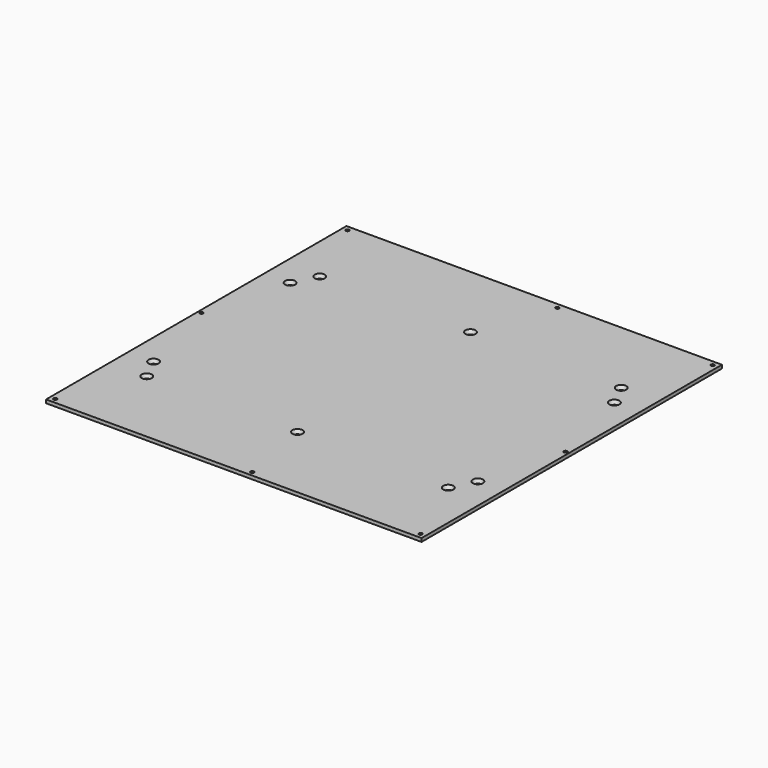
from build123d import *

# Parameters (mm, degrees)
F0_W       = 330
F0_H       = 330
F0_R       = 1.5
F0_R_2     = 2.6
F1_DEPTH   = 3
F2_SIZE2   = 1.849213
F2_SIZE    = 2.99999
F3_SIZE2   = 1.849213
F3_SIZE    = 2.99999
F3_2_SIZE2 = 1.849213
F3_2_SIZE  = 2.99999
F3_3_SIZE2 = 1.849213
F3_3_SIZE  = 2.99999
F3_4_SIZE2 = 1.849213
F3_4_SIZE  = 2.99999
F3_5_SIZE2 = 1.849213
F3_5_SIZE  = 2.99999
F3_6_SIZE2 = 1.849213
F3_6_SIZE  = 2.99999
F3_7_SIZE2 = 1.849213
F3_7_SIZE  = 2.99999
F3_8_SIZE2 = 1.849213
F3_8_SIZE  = 2.99999
F3_9_SIZE2 = 1.849213
F3_9_SIZE  = 2.99999


# Not quite as in the source:
# - a fillet or chamfer is up to 0.001 mm smaller than in the source, because OpenCascade refuses the exact size


with BuildPart() as f1:
    # F0 (on Top) → F1 (new body)
    with BuildSketch(Plane.XY):
        Rectangle(F0_W, F0_H)
        with Locations((-160.5, -160.5)):
            Circle(F0_R, mode=Mode.SUBTRACT)
        with Locations((-132.5, -95)):
            Circle(F0_R_2, mode=Mode.SUBTRACT)
        with Locations((-142.5, -75)):
            Circle(F0_R_2, mode=Mode.SUBTRACT)
        with Locations((13, -161)):
            Circle(F0_R, mode=Mode.SUBTRACT)
        with Locations((0, -95)):
            Circle(F0_R_2, mode=Mode.SUBTRACT)
        with Locations((160.5, -160.5)):
            Circle(F0_R, mode=Mode.SUBTRACT)
        with Locations((132.5, -95)):
            Circle(F0_R_2, mode=Mode.SUBTRACT)
        with Locations((142.5, -75)):
            Circle(F0_R_2, mode=Mode.SUBTRACT)
        with Locations((162, -3)):
            Circle(F0_R, mode=Mode.SUBTRACT)
        with Locations((-162, 2)):
            Circle(F0_R, mode=Mode.SUBTRACT)
        with Locations((-142.5, 75)):
            Circle(F0_R_2, mode=Mode.SUBTRACT)
        with Locations((-132.5, 95)):
            Circle(F0_R_2, mode=Mode.SUBTRACT)
        with Locations((-160.5, 160.5)):
            Circle(F0_R, mode=Mode.SUBTRACT)
        with Locations((142.5, 75)):
            Circle(F0_R_2, mode=Mode.SUBTRACT)
        with Locations((0, 95)):
            Circle(F0_R_2, mode=Mode.SUBTRACT)
        with Locations((24, 160.5)):
            Circle(F0_R, mode=Mode.SUBTRACT)
        with Locations((132.5, 95)):
            Circle(F0_R_2, mode=Mode.SUBTRACT)
        with Locations((160.5, 160.5)):
            Circle(F0_R, mode=Mode.SUBTRACT)
    extrude(amount=F1_DEPTH)

    # F2 (size 3 and 1.8492230955 in the source; OpenCascade refuses exactly that, so slightly less here)
    f2_edges = [f1.edges().sort_by_distance(p)[0] for p in [
        (-135.1, 95, 3),
    ]]
    f2_side = f1.faces().sort_by_distance((-135.1, 95, 1.5))[0]
    chamfer(f2_edges, length=F2_SIZE, length2=F2_SIZE2, reference=f2_side)

    # F3 (size 3 and 1.8492230955 in the source; OpenCascade refuses exactly that, so slightly less here)
    f3_edges = [f1.edges().sort_by_distance(p)[0] for p in [
        (-145.1, 75, 3),
    ]]
    f3_side = f1.faces().sort_by_distance((-145.1, 75, 1.5))[0]
    chamfer(f3_edges, length=F3_SIZE, length2=F3_SIZE2, reference=f3_side)

    # F3#2 (size 3 and 1.8492230955 in the source; OpenCascade refuses exactly that, so slightly less here)
    f3_2_edges = [f1.edges().sort_by_distance(p)[0] for p in [
        (-2.6, 95, 3),
    ]]
    f3_2_side = f1.faces().sort_by_distance((-2.6, 95, 1.5))[0]
    chamfer(f3_2_edges, length=F3_2_SIZE, length2=F3_2_SIZE2, reference=f3_2_side)

    # F3#3 (size 3 and 1.8492230955 in the source; OpenCascade refuses exactly that, so slightly less here)
    f3_3_edges = [f1.edges().sort_by_distance(p)[0] for p in [
        (129.9, 95, 3),
    ]]
    f3_3_side = f1.faces().sort_by_distance((129.9, 95, 1.5))[0]
    chamfer(f3_3_edges, length=F3_3_SIZE, length2=F3_3_SIZE2, reference=f3_3_side)

    # F3#4 (size 3 and 1.8492230955 in the source; OpenCascade refuses exactly that, so slightly less here)
    f3_4_edges = [f1.edges().sort_by_distance(p)[0] for p in [
        (139.9, 75, 3),
    ]]
    f3_4_side = f1.faces().sort_by_distance((139.9, 75, 1.5))[0]
    chamfer(f3_4_edges, length=F3_4_SIZE, length2=F3_4_SIZE2, reference=f3_4_side)

    # F3#5 (size 3 and 1.8492230955 in the source; OpenCascade refuses exactly that, so slightly less here)
    f3_5_edges = [f1.edges().sort_by_distance(p)[0] for p in [
        (139.9, -75, 3),
    ]]
    f3_5_side = f1.faces().sort_by_distance((139.9, -75, 1.5))[0]
    chamfer(f3_5_edges, length=F3_5_SIZE, length2=F3_5_SIZE2, reference=f3_5_side)

    # F3#6 (size 3 and 1.8492230955 in the source; OpenCascade refuses exactly that, so slightly less here)
    f3_6_edges = [f1.edges().sort_by_distance(p)[0] for p in [
        (129.9, -95, 3),
    ]]
    f3_6_side = f1.faces().sort_by_distance((129.9, -95, 1.5))[0]
    chamfer(f3_6_edges, length=F3_6_SIZE, length2=F3_6_SIZE2, reference=f3_6_side)

    # F3#7 (size 3 and 1.8492230955 in the source; OpenCascade refuses exactly that, so slightly less here)
    f3_7_edges = [f1.edges().sort_by_distance(p)[0] for p in [
        (-2.6, -95, 3),
    ]]
    f3_7_side = f1.faces().sort_by_distance((-2.6, -95, 1.5))[0]
    chamfer(f3_7_edges, length=F3_7_SIZE, length2=F3_7_SIZE2, reference=f3_7_side)

    # F3#8 (size 3 and 1.8492230955 in the source; OpenCascade refuses exactly that, so slightly less here)
    f3_8_edges = [f1.edges().sort_by_distance(p)[0] for p in [
        (-135.1, -95, 3),
    ]]
    f3_8_side = f1.faces().sort_by_distance((-135.1, -95, 1.5))[0]
    chamfer(f3_8_edges, length=F3_8_SIZE, length2=F3_8_SIZE2, reference=f3_8_side)

    # F3#9 (size 3 and 1.8492230955 in the source; OpenCascade refuses exactly that, so slightly less here)
    f3_9_edges = [f1.edges().sort_by_distance(p)[0] for p in [
        (-145.1, -75, 3),
    ]]
    f3_9_side = f1.faces().sort_by_distance((-145.1, -75, 1.5))[0]
    chamfer(f3_9_edges, length=F3_9_SIZE, length2=F3_9_SIZE2, reference=f3_9_side)


solid = f1.part
